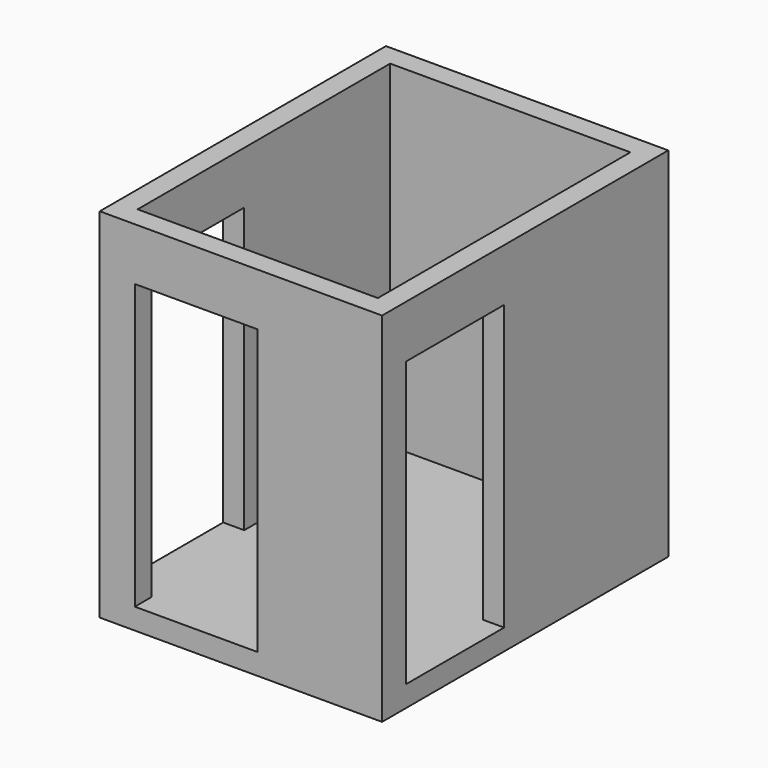
from build123d import *

# Parameters (mm, degrees)
F1_DEPTH = 2438.4
F2_START = 2057.4
F0_W     = 152.4
F0_H     = 889
F0_W_2   = 889
F0_H_2   = 152.4
F2_DEPTH = 381
F0_W_3   = 101.6
F0_H_3   = 76.2
F3_DEPTH = 152.4


with BuildPart() as f1:
    # F0 (on Top) → F1 (new body)
    with BuildSketch(Plane.XY):
        Polygon((-152.4, 965.2), (0, 965.2), (0, 2286), (1739.9, 2286), (1739.9, 952.5), (1892.3, 952.5), (1892.3, 2438.4), (-152.4, 2438.4), align=None)
    extrude(amount=F1_DEPTH)



with BuildPart() as f1b:
    # F0 (on Top) → F1, piece 2 (new body)
    with BuildSketch(Plane.XY):
        Polygon((1739.9, 0), (990.6, 0), (990.6, -152.4), (1892.3, -152.4), (1892.3, 63.5), (1739.9, 63.5), align=None)
    extrude(amount=F1_DEPTH)


with BuildPart() as f1c:
    # F0 (on Top) → F1, piece 3 (new body)
    with BuildSketch(Plane.XY):
        Polygon((101.6, 0), (0, 0), (0, 76.2), (-152.4, 76.2), (-152.4, -152.4), (101.6, -152.4), align=None)
    extrude(amount=F1_DEPTH)


with BuildPart() as f1_1:
    add(f1.part)

    add(f1b.part)  # F2 merges F1b

    add(f1c.part)  # F2 merges F1c
    # F0 (on Top) → F2 (join)
    with BuildSketch(Plane.XY.offset(F2_START)):
        with Locations((-76.2, 520.7)):
            Rectangle(F0_W, F0_H)
        with Locations((1816.1, 508)):
            Rectangle(F0_W, F0_H)
        with Locations((546.1, -76.2)):
            Rectangle(F0_W_2, F0_H_2)
    extrude(amount=F2_DEPTH)

    # F0 (on Top) → F3 (join)
    with BuildSketch(Plane.XY):
        Polygon((101.6, 0), (0, 0), (0, 76.2), (-152.4, 76.2), (-152.4, -152.4), (101.6, -152.4), align=None)
        with Locations((546.1, -76.2)):
            Rectangle(F0_W_2, F0_H_2)
        with Locations((-76.2, 520.7)):
            Rectangle(F0_W, F0_H)
        Polygon((1739.9, 0), (990.6, 0), (990.6, -152.4), (1892.3, -152.4), (1892.3, 63.5), (1739.9, 63.5), align=None)
        Polygon((-152.4, 965.2), (0, 965.2), (0, 2286), (1739.9, 2286), (1739.9, 952.5), (1892.3, 952.5), (1892.3, 2438.4), (-152.4, 2438.4), align=None)
        with Locations((1816.1, 508)):
            Rectangle(F0_W, F0_H)
        with BuildLine():
            ThreePointArc((850.9, 952.5), (1111.2820715252, 323.8820715252), (1739.9, 63.5))
            Line((1739.9, 63.5), (1739.9, 952.5))
            Line((1739.9, 952.5), (850.9, 952.5))
        make_face()
        with BuildLine():
            ThreePointArc((582.8375456676, 747.4833942235), (882.0297463893, 425.7351417851), (990.6, 0))
            Line((990.6, 0), (1739.9, 0))
            Line((1739.9, 0), (1739.9, 63.5))
            ThreePointArc((1739.9, 63.5), (1111.2820715252, 323.8820715252), (850.9, 952.5))
            Line((850.9, 952.5), (1739.9, 952.5))
            Line((1739.9, 952.5), (1739.9, 2286))
            Line((1739.9, 2286), (0, 2286))
            Line((0, 2286), (0, 965.2))
            ThreePointArc((0, 965.2), (311.0868548616, 908.9940734253), (582.8375456676, 747.4833942235))
        make_face()
        with BuildLine():
            Line((101.6, 889), (101.6, 76.2))
            Line((101.6, 76.2), (889, 76.2))
            ThreePointArc((889, 76.2), (808.8459612616, 445.1027120404), (582.8375456676, 747.4833942235))
            ThreePointArc((582.8375456676, 747.4833942235), (352.4069601659, 852.8873716572), (101.6, 889))
        make_face()
        with BuildLine():
            Line((0, 965.2), (0, 76.2))
            Line((0, 76.2), (101.6, 76.2))
            Line((101.6, 76.2), (101.6, 889))
            ThreePointArc((101.6, 889), (352.4069601659, 852.8873716572), (582.8375456676, 747.4833942235))
            ThreePointArc((582.8375456676, 747.4833942235), (311.0868548616, 908.9940734253), (0, 965.2))
        make_face()
        with BuildLine():
            Line((101.6, 76.2), (101.6, 0))
            Line((101.6, 0), (990.6, 0))
            ThreePointArc((990.6, 0), (882.0297463893, 425.7351417851), (582.8375456676, 747.4833942235))
            ThreePointArc((582.8375456676, 747.4833942235), (808.8459612616, 445.1027120404), (889, 76.2))
            Line((889, 76.2), (101.6, 76.2))
        make_face()
        with Locations((50.8, 38.1)):
            Rectangle(F0_W_3, F0_H_3)
    extrude(amount=-F3_DEPTH)


solid = f1_1.part
